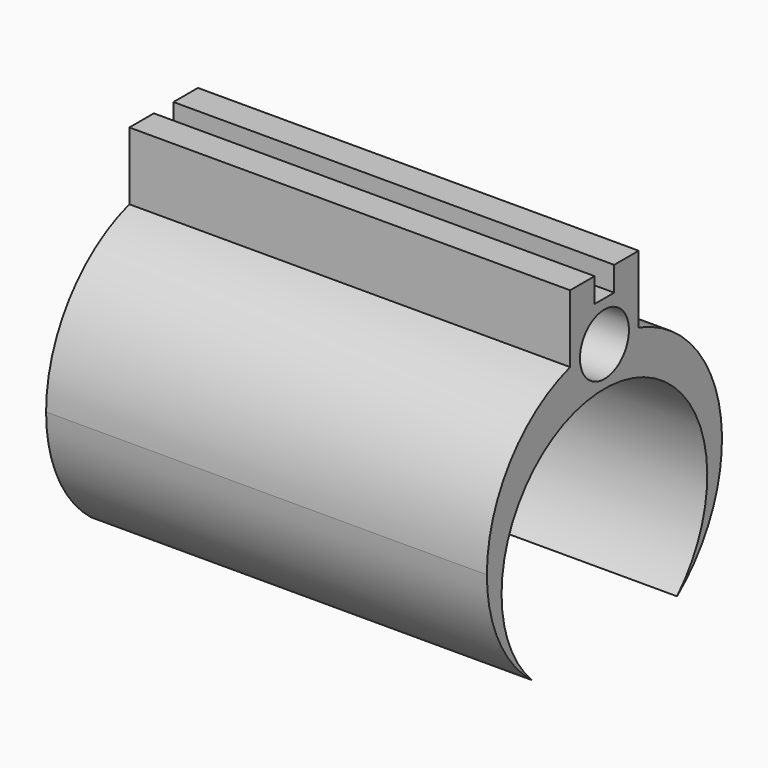
from build123d import *

# Parameters (mm, degrees)
F0_W     = 18
F0_H     = 3.5
F1_DEPTH = 2.5
F3_DEPTH = 1
F4_W     = 18
F4_H     = 3.5
F5_DEPTH = 0.5
F7_DEPTH = 18
F8_R     = 1.25
F9_DEPTH = 18.001


with BuildPart() as f1:
    # F0 (on Top) → F1 (new body)
    with BuildSketch(Plane.XY):
        Rectangle(F0_W, F0_H)
    extrude(amount=F1_DEPTH)

    # F2 (on face) → F3 (cut)
    with BuildSketch(Plane.XY.offset(2.5)):
        with BuildLine():
            ThreePointArc((-8.5, 0), (-8.6464466094, 0.3535533906), (-9, 0.5))
            Line((-9, 0.5), (-9, -0.5))
            ThreePointArc((-9, -0.5), (-8.6464466094, -0.3535533906), (-8.5, 0))
        make_face()
        with BuildLine():
            Line((9, 0.5), (-9, 0.5))
            ThreePointArc((-9, 0.5), (-8.6464466094, 0.3535533906), (-8.5, 0))
            ThreePointArc((-8.5, 0), (-8.6464466094, -0.3535533906), (-9, -0.5))
            Line((-9, -0.5), (9, -0.5))
            ThreePointArc((9, -0.5), (8.5, 0), (9, 0.5))
        make_face()
        with BuildLine():
            Line((-9, -0.5), (-9, 0.5))
            ThreePointArc((-9, 0.5), (-9.5, 0), (-9, -0.5))
        make_face()
        with BuildLine():
            ThreePointArc((9.5, 0), (9.3535533906, 0.3535533906), (9, 0.5))
            Line((9, 0.5), (9, -0.5))
            ThreePointArc((9, -0.5), (9.3535533906, -0.3535533906), (9.5, 0))
        make_face()
        with BuildLine():
            Line((9, -0.5), (9, 0.5))
            ThreePointArc((9, 0.5), (8.5, 0), (9, -0.5))
        make_face()
    extrude(amount=-F3_DEPTH, mode=Mode.SUBTRACT)

    # F4 (on face) → F5 (join)
    with BuildSketch(Plane(origin=(0, 0, 0), x_dir=(1, 0, 0), z_dir=(0, 0, -1))):
        Rectangle(F4_W, F4_H)
    extrude(amount=F5_DEPTH)

    # F6 (on face) → F7 (join)
    with BuildSketch(Plane(origin=(-9, 0, 0), x_dir=(0, -1, 0), z_dir=(-1, 0, 0))):
        with BuildLine():
            ThreePointArc((3.7058600132, -10.71875), (5.3960707964, -8.6234366698), (6, -6))
            ThreePointArc((6, -6), (4.8218253805, -2.4292857857), (1.75, -0.2608798584))
            Line((1.75, -0.2608798584), (1.75, -0.5))
            Line((1.75, -0.5), (-1.75, -0.5))
            Line((-1.75, -0.5), (-1.75, -0.2608798584))
            ThreePointArc((-1.75, -0.2608798584), (-5.897742288, -4.8969878041), (-3.7058600132, -10.71875))
            ThreePointArc((-3.7058600132, -10.71875), (-2.0132976594, -2.1513782851), (5.25, -7))
            ThreePointArc((5.25, -7), (4.8486217149, -9.0132976594), (3.7058600132, -10.71875))
        make_face()
        with BuildLine():
            Line((1.75, -0.5), (1.75, -0.2608798584))
            ThreePointArc((1.75, -0.2608798584), (0, 0), (-1.75, -0.2608798584))
            Line((-1.75, -0.2608798584), (-1.75, -0.5))
            Line((-1.75, -0.5), (1.75, -0.5))
        make_face()
    extrude(amount=-F7_DEPTH)

    # F8 (on face) → F9 (cut, through all)
    with BuildSketch(Plane.YZ.offset(9)):
        with Locations((0, -0.15)):
            Circle(F8_R)
    extrude(amount=-F9_DEPTH, mode=Mode.SUBTRACT)


solid = f1.part
